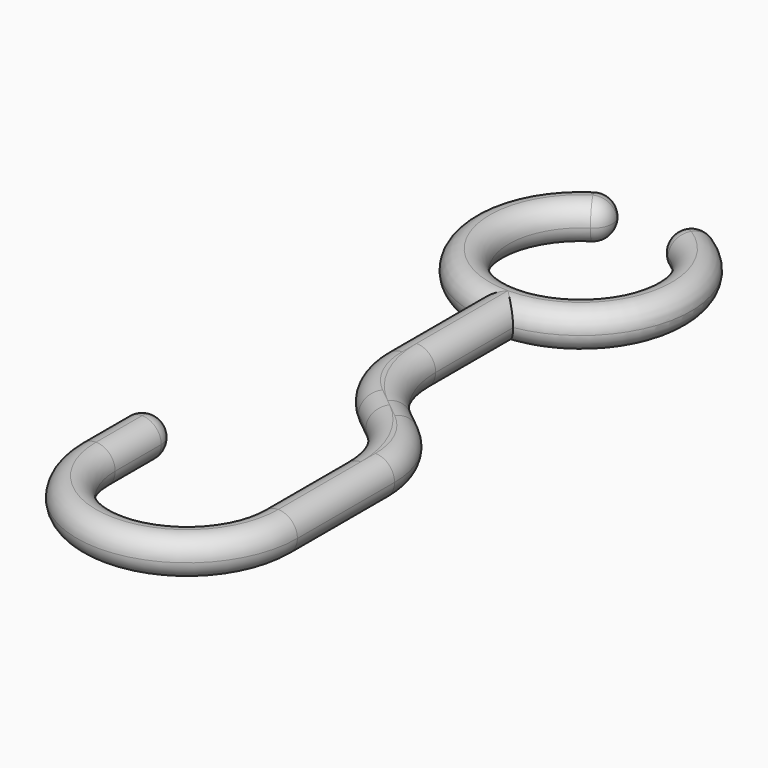
from build123d import *

# Parameters (mm, degrees)
F1_DEPTH = 4
F2_R     = 1.99999


# Not quite as in the source:
# - a fillet or chamfer is up to 0.001 mm smaller than in the source, because OpenCascade refuses the exact size


with BuildPart() as f1:
    # F0 (on Top) → F1 (new body)
    with BuildSketch(Plane.XY):
        with BuildLine():
            ThreePointArc((4.0480979968, 6.3137075168), (0, -7.5), (-4.0480979968, 6.3137075168))
            ThreePointArc((-4.0480979968, 6.3137075168), (-3.2081276873, 7.4355253564), (-3.310625946, 8.8332089733))
            ThreePointArc((-3.310625946, 8.8332089733), (-4.5657532977, 9.9168259633), (-6.2070835951, 9.6810181925))
            ThreePointArc((-6.2070835951, 9.6810181925), (-11.2760652261, -2.2583961159), (-2, -11.3247516529))
            Line((-2, -11.3247516529), (-2, -23.3247516529))
            ThreePointArc((-2, -23.3247516529), (-1.0269337206, -27.6275957825), (1.7028935206, -31.0930494064))
            Line((1.7028935206, -31.0930494064), (3.7971064794, -32.7906519456))
            ThreePointArc((3.7971064794, -32.7906519456), (6.5269337206, -36.2561055696), (7.5, -40.5589496992))
            Line((7.5, -40.5589496992), (7.5, -51.3247516529))
            ThreePointArc((7.5, -51.3247516529), (0, -58.8247516529), (-7.5, -51.3247516529))
            Line((-7.5, -51.3247516529), (-7.5, -45.3247516529))
            ThreePointArc((-7.5, -45.3247516529), (-8.0857864376, -43.9105380905), (-9.5, -43.3247516529))
            ThreePointArc((-9.5, -43.3247516529), (-10.9142135624, -43.9105380905), (-11.5, -45.3247516529))
            Line((-11.5, -45.3247516529), (-11.5, -51.3247516529))
            ThreePointArc((-11.5, -51.3247516529), (0, -62.8247516529), (11.5, -51.3247516529))
            Line((11.5, -51.3247516529), (11.5, -38.6522804967))
            ThreePointArc((11.5, -38.6522804967), (10.5269337206, -34.3494363671), (7.7971064794, -30.8839827431))
            Line((7.7971064794, -30.8839827431), (5.7028935206, -29.1863802039))
            ThreePointArc((5.7028935206, -29.1863802039), (2.9730662794, -25.72092658), (2, -21.4180824504))
            Line((2, -21.4180824504), (2, -11.3247516529))
            ThreePointArc((2, -11.3247516529), (11.2760652261, -2.2583961159), (6.2070835951, 9.6810181925))
            ThreePointArc((6.2070835951, 9.6810181925), (4.5657532977, 9.9168259633), (3.310625946, 8.8332089733))
            ThreePointArc((3.310625946, 8.8332089733), (3.2081276873, 7.4355253564), (4.0480979968, 6.3137075168))
        make_face()
    extrude(amount=F1_DEPTH)

    # F2 (radius 2 in the source; OpenCascade refuses exactly that, so slightly less here)
    f2_edges = [f1.edges().sort_by_distance(p)[0] for p in [
        (-11.5, -48.324752, 4),
        (0, -62.824752, 4),
        (11.5, -44.988516, 4),
        (10.526934, -34.349436, 4),
        (6.75, -30.035181, 4),
        (2.973066, -25.720927, 4),
        (2, -16.371417, 4),
        (11.276065, -2.258396, 4),
        (3.443935, 9.076856, 4),
        (0, -7.5, 4),
        (-3.443935, 9.076856, 4),
        (-11.276065, -2.258396, 4),
        (-2, -17.324752, 4),
        (-1.026934, -27.627596, 4),
        (2.75, -31.941851, 4),
        (6.526934, -36.256106, 4),
        (7.5, -45.941851, 4),
        (0, -58.824752, 4),
        (-7.5, -48.324752, 4),
        (-9.5, -43.324752, 4),
        (-11.5, -48.324752, 0),
        (0, -62.824752, 0),
        (11.5, -44.988516, 0),
        (10.526934, -34.349436, 0),
        (6.75, -30.035181, 0),
        (2.973066, -25.720927, 0),
        (2, -16.371417, 0),
        (11.276065, -2.258396, 0),
        (3.443935, 9.076856, 0),
        (0, -7.5, 0),
        (-3.443935, 9.076856, 0),
        (-11.276065, -2.258396, 0),
        (-2, -17.324752, 0),
        (-1.026934, -27.627596, 0),
        (2.75, -31.941851, 0),
        (6.526934, -36.256106, 0),
        (7.5, -45.941851, 0),
        (0, -58.824752, 0),
        (-7.5, -48.324752, 0),
        (-9.5, -43.324752, 0),
    ]]
    fillet(f2_edges, radius=F2_R)


solid = f1.part
